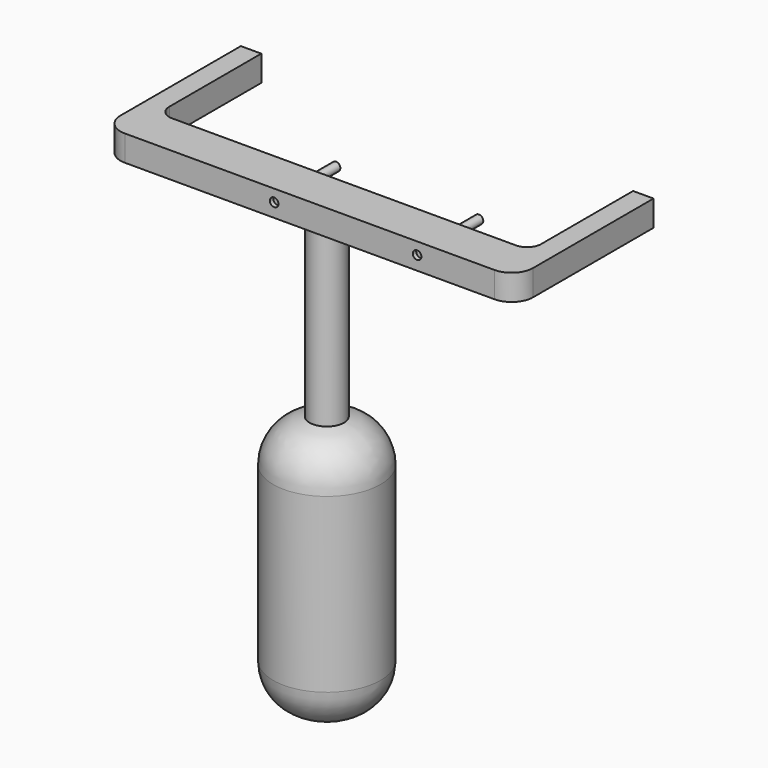
from build123d import *

# Parameters (mm, degrees)
F1_DEPTH  = 6
F2_R      = 3.25
F3_R      = 5
F4_R      = 1
F5_DEPTH  = 10
F6_R      = 4
F7_DEPTH  = 40
F8_R      = 12.5
F8_R_2    = 4
F9_DEPTH  = 60
F12_R     = 1
F13_DEPTH = 17


# Not quite as in the source:
# - a fillet or chamfer that OpenCascade refuses, or shapes differently, is made with other operations: its cross-section is extruded or revolved along the edge and cut away or added


with BuildPart() as f1:
    # F0 (on Top) → F1 (new body)
    with BuildSketch(Plane.XY):
        Polygon((-48, -5), (-48, -45), (48, -45), (48, -5), (43.25, -5), (43.25, -35), (-43.25, -35), (-43.25, -5), align=None)
    extrude(amount=F1_DEPTH)

    # F2
    f2_edges = [f1.edges().sort_by_distance(p)[0] for p in [
        (-43.25, -35, 3),
        (43.25, -35, 3),
    ]]
    fillet(f2_edges, radius=F2_R)

    # F3
    f3_edges = [f1.edges().sort_by_distance(p)[0] for p in [
        (48, -45, 3),
        (-48, -45, 3),
    ]]
    fillet(f3_edges, radius=F3_R)

    # F4 (on face) → F5 (cut)
    with BuildSketch(Plane.XZ.offset(45)):
        with Locations((-8.25, 3.2)):
            Circle(F4_R)
        with Locations((25, 3.2)):
            Circle(F4_R)
    extrude(amount=-F5_DEPTH, mode=Mode.SUBTRACT)

    # F6 (on face) → F7 (join)
    with BuildSketch(Plane(origin=(0, 0, 0), x_dir=(1, 0, 0), z_dir=(0, 0, -1))):
        with Locations((0, 40)):
            Circle(F6_R)
    extrude(amount=F7_DEPTH)

    # F8 (on face) → F9 (join)
    with BuildSketch(Plane(origin=(0, 0, -40), x_dir=(1, 0, 0), z_dir=(0, 0, -1))):
        with Locations((0, 40)):
            Circle(F8_R)
        with Locations((0, 40)):
            Circle(F8_R_2, mode=Mode.SUBTRACT)
        with Locations((0, 40)):
            Circle(F8_R_2)
    extrude(amount=F9_DEPTH)

    # F10: fillet of radius 10 on 2 edges, made by hand

    # F10_s1 → F10_t2 (revolve, cut)
    with BuildSketch(Plane.XZ.offset(40)):
        with BuildLine():
            ThreePointArc((12.5, -90), (9.5710678119, -97.0710678119), (2.5, -100))
            Line((2.5, -100), (12.5, -100))
            Line((12.5, -100), (12.5, -90))
        make_face()
    revolve(axis=Axis((0, -40, -100), (0, 0, -1)), mode=Mode.SUBTRACT)

    # F10_s3 → F10_t4 (revolve, cut)
    with BuildSketch(Plane.XZ.offset(40)):
        with BuildLine():
            ThreePointArc((12.5, -49.8868599666), (10.0828754441, -43.3676575614), (4, -40))
            Line((4, -40), (12.5, -40))
            Line((12.5, -40), (12.5, -49.8868599666))
        make_face()
    revolve(axis=Axis((0, -40, -40), (0, 0, -1)), mode=Mode.SUBTRACT)

    # F12 (on offset) → F13 (join)
    with BuildSketch(Plane.XZ.offset(44)):
        with Locations((-8.25, 3.2)):
            Circle(F12_R)
        with Locations((25, 3.2)):
            Circle(F12_R)
    extrude(amount=-F13_DEPTH)


solid = f1.part
